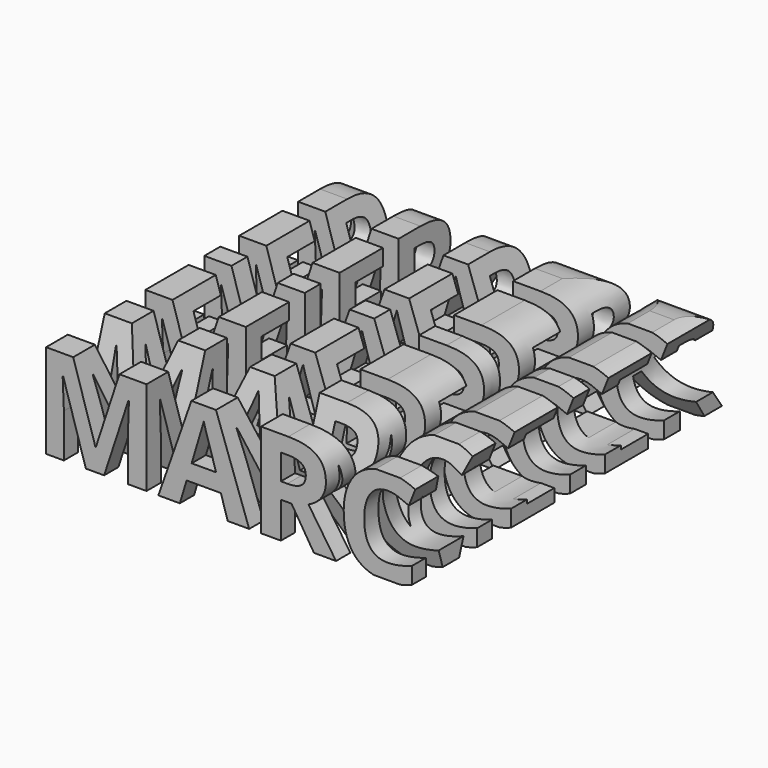
from build123d import *

# Parameters (mm, degrees)
F0_TEXT_SIZE = 83.3333333333
F1_DEPTH     = 200
F2_TEXT_SIZE = 83.3333333333
F3_DEPTH     = 250


# Not quite as in the source:
# - Text() gives the source's letters only with a copy of the font that has no kerning and outlines rounded to 1/6400 em; it was checked with that copy


with BuildPart() as f1:
    # F0 (on Front) → F1 (new body, symmetric)
    with BuildSketch(Plane.XZ):
        with Locations((-123.3268229167, -30)):
            Text('MARC', F0_TEXT_SIZE, font='Open Sans', font_style=FontStyle.BOLD, text_align=(TextAlign.LEFT, TextAlign.BOTTOM))
    extrude(amount=F1_DEPTH, both=True)

    # F2 (on Right) → F3 (intersect, symmetric)
    with BuildSketch(Plane.YZ):
        with Locations((-129.9544270833, -30)):
            Text('MEIER', F2_TEXT_SIZE, font='Open Sans', font_style=FontStyle.BOLD, text_align=(TextAlign.LEFT, TextAlign.BOTTOM))
    extrude(amount=F3_DEPTH, both=True, mode=Mode.INTERSECT)


solid = f1.part
